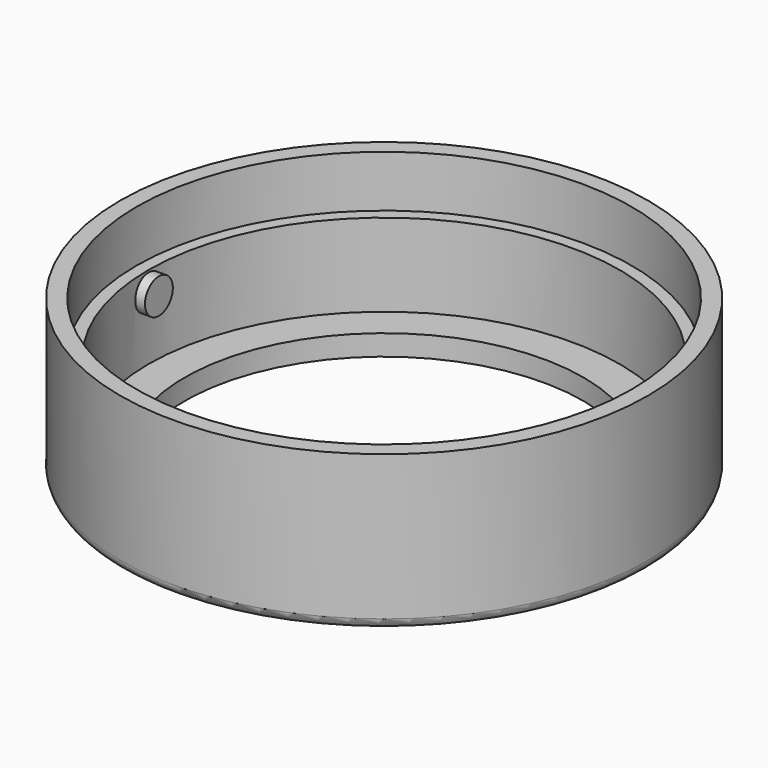
from build123d import *

# Parameters (mm, degrees)
F0_R     = 22.75
F0_R_2   = 19.25
F1_DEPTH = 2
F0_R_3   = 23.9
F2_DEPTH = 10
F0_R_4   = 25.5
F3_DEPTH = 15
F6_DEPTH = 2
F7_R     = 1


# Not quite as in the source:
# - a pattern or mirror of a feature is missing from the dataset's text; its kind, count and spacing are read off the source's solid


with BuildPart() as f1:
    # F0 (on Top) → F1 (new body)
    with BuildSketch(Plane.XY):
        Circle(F0_R)
        Circle(F0_R_2, mode=Mode.SUBTRACT)
    extrude(amount=F1_DEPTH)


with BuildPart() as f2:
    # F0 (on Top) → F2 (new body)
    with BuildSketch(Plane.XY):
        Circle(F0_R_3)
        Circle(F0_R, mode=Mode.SUBTRACT)
    extrude(amount=F2_DEPTH)

    # F0 (on Top) → F3 (join)
    with BuildSketch(Plane.XY):
        Circle(F0_R_4)
        Circle(F0_R_3, mode=Mode.SUBTRACT)
    extrude(amount=F3_DEPTH)

    # F5 (on offset) → F6 (join)
    with BuildSketch(Plane.YZ.offset(21.75)):
        with BuildLine():
            ThreePointArc((0, 6.4177232337), (1.1895493093, 6.9104506907), (1.6822767663, 8.1))
            ThreePointArc((1.6822767663, 8.1), (-1.1895493093, 9.2895493093), (0, 6.4177232337))
        make_face()
    f6 = extrude(amount=F6_DEPTH)

    # F6_copies: F6 across plane
    add(f6.mirror(Plane(origin=(0, 0, 0), x_dir=(0, 0, -1), z_dir=(-1, 0, 0))))

    # F7
    f7_edges = [f2.edges().sort_by_distance(p)[0] for p in [
        (-25.5, 0, 0),
    ]]
    fillet(f7_edges, radius=F7_R)


solid = Compound([f1.part, f2.part])
